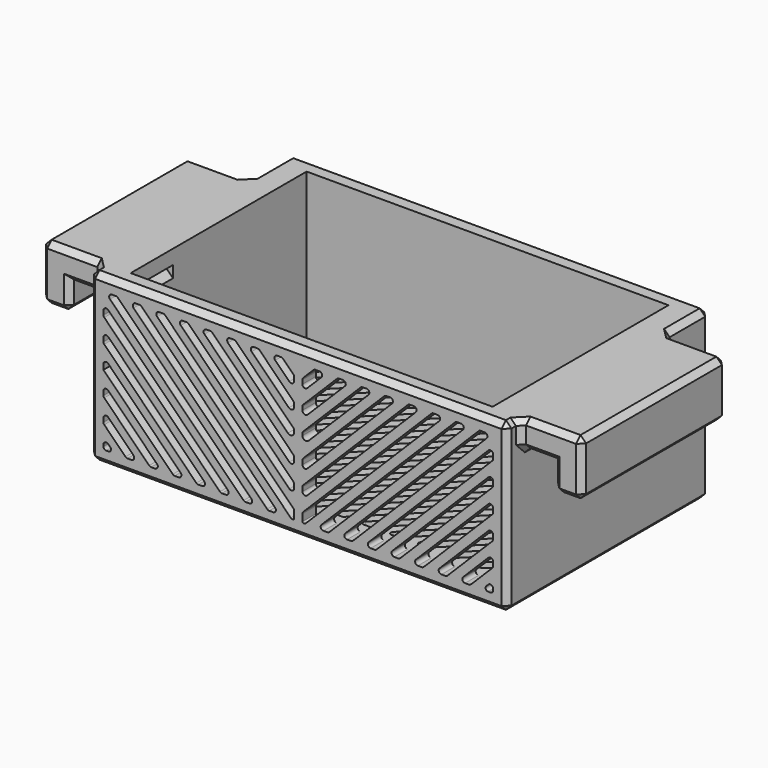
from build123d import *

# Parameters (mm, degrees)
F0_W          = 10
F0_H          = 65
F1_DEPTH      = 10
F1_DEPTH_BACK = 10
F0_W_2        = 12
F2_DEPTH      = 10
F3_DEPTH      = 10
F3_DEPTH_BACK = 50
F4_DEPTH      = 10
F4_DEPTH_BACK = 50
F0_W_3        = 130
F0_H_2        = 6
F5_DEPTH      = 10
F5_DEPTH_BACK = 50
F6_START      = -45
F0_H_3        = 79
F6_DEPTH      = 5
F8_DEPTH      = 58.3
F9_SIZE       = 2
F11_DEPTH     = 25
F12_DEPTH     = 25


with BuildPart() as f1:
    # F0 (on Top) → F1 (new body, two sides)
    with BuildSketch(Plane.XY) as f1_sk:
        with Locations((-167, -32.5)):
            Rectangle(F0_W, F0_H)
    extrude(amount=-F1_DEPTH)
    extrude(f1_sk.sketch, amount=F1_DEPTH_BACK)

    # F0 (on Top) → F2 (join)
    with BuildSketch(Plane.XY):
        with Locations((-156, -32.5)):
            Rectangle(F0_W_2, F0_H)
    extrude(amount=F2_DEPTH)

    # F0 (on Top) → F3 (join, two sides)
    with BuildSketch(Plane.XY) as f3_sk:
        Polygon((-150, -65), (-140, -65), (-140, 14), (-140, 20), (-150, 20), (-150, 0), align=None)
    extrude(amount=F3_DEPTH)
    extrude(f3_sk.sketch, amount=-F3_DEPTH_BACK)



with BuildPart() as f1b:
    # F0 (on Top) → F1, piece 2 (new body, two sides)
    with BuildSketch(Plane.XY) as f1_2_sk:
        with Locations((17, -32.5)):
            Rectangle(F0_W, F0_H)
    extrude(amount=-F1_DEPTH)
    extrude(f1_2_sk.sketch, amount=F1_DEPTH_BACK)

    # F0 (on Top) → F2, piece 2 (join)
    with BuildSketch(Plane.XY):
        with Locations((6, -32.5)):
            Rectangle(F0_W_2, F0_H)
    extrude(amount=F2_DEPTH)

    # F0 (on Top) → F3, piece 2 (join, two sides)
    with BuildSketch(Plane.XY) as f3_2_sk:
        Polygon((0, -65), (0, 0), (0, 20), (-10, 20), (-10, 14), (-10, -65), align=None)
    extrude(amount=F3_DEPTH)
    extrude(f3_2_sk.sketch, amount=-F3_DEPTH_BACK)


with BuildPart() as f1_1:
    add(f1.part)

    add(f1b.part)  # F4 merges F1b
    # F0 (on Top) → F4 (join, two sides)
    with BuildSketch(Plane.XY) as f4_sk:
        Polygon((0, -71), (0, -65), (-10, -65), (-140, -65), (-150, -65), (-150, -71), align=None)
    extrude(amount=F4_DEPTH)
    extrude(f4_sk.sketch, amount=-F4_DEPTH_BACK)

    # F0 (on Top) → F5 (join, two sides)
    with BuildSketch(Plane.XY) as f5_sk:
        with Locations((-75, 17)):
            Rectangle(F0_W_3, F0_H_2)
    extrude(amount=F5_DEPTH)
    extrude(f5_sk.sketch, amount=-F5_DEPTH_BACK)

    # F0 (on Top) → F6 (join)
    with BuildSketch(Plane.XY.offset(F6_START)):
        with Locations((-75, -25.5)):
            Rectangle(F0_W_3, F0_H_3)
    extrude(amount=-F6_DEPTH)

    # F7 (on face) → F8 (cut)
    with BuildSketch(Plane.XY):
        with BuildLine():
            Line((-131, 10), (-136, 5))
            Line((-136, 5), (-136, 2.4142135624))
            ThreePointArc((-136, 2.4142135624), (-135.3826834324, 1.4903340299), (-134.2928932188, 1.7071067812))
            Line((-134.2928932188, 1.7071067812), (-127.7071067812, 8.2928932188))
            ThreePointArc((-127.7071067812, 8.2928932188), (-127.4903340299, 9.3826834324), (-128.4142135624, 10))
            Line((-128.4142135624, 10), (-131, 10))
        make_face()
        with BuildLine():
            Line((-121.2928932188, 9.7071067812), (-135.7071067812, -4.7071067812))
            ThreePointArc((-135.7071067812, -4.7071067812), (-135.9238795325, -5.03153013), (-136, -5.4142135624))
            Line((-136, -5.4142135624), (-136, -7.5857864376))
            ThreePointArc((-136, -7.5857864376), (-135.3826834324, -8.5096659701), (-134.2928932188, -8.2928932188))
            Line((-134.2928932188, -8.2928932188), (-117.7071067812, 8.2928932188))
            ThreePointArc((-117.7071067812, 8.2928932188), (-117.4903340299, 9.3826834324), (-118.4142135624, 10))
            Line((-118.4142135624, 10), (-120.5857864376, 10))
            ThreePointArc((-120.5857864376, 10), (-120.96846987, 9.9238795325), (-121.2928932188, 9.7071067812))
        make_face()
        with BuildLine():
            Line((-111.2928932188, 9.7071067812), (-135.7071067812, -14.7071067812))
            ThreePointArc((-135.7071067812, -14.7071067812), (-135.9238795325, -15.03153013), (-136, -15.4142135624))
            Line((-136, -15.4142135624), (-136, -17.5857864376))
            ThreePointArc((-136, -17.5857864376), (-135.3826834324, -18.5096659701), (-134.2928932188, -18.2928932188))
            Line((-134.2928932188, -18.2928932188), (-107.7071067812, 8.2928932188))
            ThreePointArc((-107.7071067812, 8.2928932188), (-107.4903340299, 9.3826834324), (-108.4142135624, 10))
            Line((-108.4142135624, 10), (-110.5857864376, 10))
            ThreePointArc((-110.5857864376, 10), (-110.96846987, 9.9238795325), (-111.2928932188, 9.7071067812))
        make_face()
        with BuildLine():
            Line((-101.2928932188, 9.7071067812), (-135.7071067812, -24.7071067812))
            ThreePointArc((-135.7071067812, -24.7071067812), (-135.9238795325, -25.03153013), (-136, -25.4142135624))
            Line((-136, -25.4142135624), (-136, -27.5857864376))
            ThreePointArc((-136, -27.5857864376), (-135.3826834324, -28.5096659701), (-134.2928932188, -28.2928932188))
            Line((-134.2928932188, -28.2928932188), (-97.7071067812, 8.2928932188))
            ThreePointArc((-97.7071067812, 8.2928932188), (-97.4903340299, 9.3826834324), (-98.4142135624, 10))
            Line((-98.4142135624, 10), (-100.5857864376, 10))
            ThreePointArc((-100.5857864376, 10), (-100.96846987, 9.9238795325), (-101.2928932188, 9.7071067812))
        make_face()
        with BuildLine():
            Line((-91.2928932188, 9.7071067812), (-135.7071067812, -34.7071067812))
            ThreePointArc((-135.7071067812, -34.7071067812), (-135.9238795325, -35.03153013), (-136, -35.4142135624))
            Line((-136, -35.4142135624), (-136, -37.5857864376))
            ThreePointArc((-136, -37.5857864376), (-135.3826834324, -38.5096659701), (-134.2928932188, -38.2928932188))
            Line((-134.2928932188, -38.2928932188), (-87.7071067812, 8.2928932188))
            ThreePointArc((-87.7071067812, 8.2928932188), (-87.4903340299, 9.3826834324), (-88.4142135624, 10))
            Line((-88.4142135624, 10), (-90.5857864376, 10))
            ThreePointArc((-90.5857864376, 10), (-90.96846987, 9.9238795325), (-91.2928932188, 9.7071067812))
        make_face()
        with BuildLine():
            Line((-81.2928932188, 9.7071067812), (-135.7071067812, -44.7071067812))
            ThreePointArc((-135.7071067812, -44.7071067812), (-135.9238795325, -45.03153013), (-136, -45.4142135624))
            Line((-136, -45.4142135624), (-136, -47.5857864376))
            ThreePointArc((-136, -47.5857864376), (-135.3826834324, -48.5096659701), (-134.2928932188, -48.2928932188))
            Line((-134.2928932188, -48.2928932188), (-77.7071067812, 8.2928932188))
            ThreePointArc((-77.7071067812, 8.2928932188), (-77.4903340299, 9.3826834324), (-78.4142135624, 10))
            Line((-78.4142135624, 10), (-80.5857864376, 10))
            ThreePointArc((-80.5857864376, 10), (-80.96846987, 9.9238795325), (-81.2928932188, 9.7071067812))
        make_face()
        with BuildLine():
            Line((-71.2928932188, 9.7071067812), (-135.7071067812, -54.7071067812))
            ThreePointArc((-135.7071067812, -54.7071067812), (-135.9238795325, -55.03153013), (-136, -55.4142135624))
            Line((-136, -55.4142135624), (-136, -57.5857864376))
            ThreePointArc((-136, -57.5857864376), (-135.3826834324, -58.5096659701), (-134.2928932188, -58.2928932188))
            Line((-134.2928932188, -58.2928932188), (-67.7071067812, 8.2928932188))
            ThreePointArc((-67.7071067812, 8.2928932188), (-67.4903340299, 9.3826834324), (-68.4142135624, 10))
            Line((-68.4142135624, 10), (-70.5857864376, 10))
            ThreePointArc((-70.5857864376, 10), (-70.96846987, 9.9238795325), (-71.2928932188, 9.7071067812))
        make_face()
        with BuildLine():
            ThreePointArc((-130.2928932188, -59.2928932188), (-130.5096659701, -60.3826834324), (-129.5857864376, -61))
            Line((-129.5857864376, -61), (-127.4142135624, -61))
            ThreePointArc((-127.4142135624, -61), (-127.03153013, -60.9238795325), (-126.7071067812, -60.7071067812))
            Line((-126.7071067812, -60.7071067812), (-57.7071067812, 8.2928932188))
            ThreePointArc((-57.7071067812, 8.2928932188), (-57.4903340299, 9.3826834324), (-58.4142135624, 10))
            Line((-58.4142135624, 10), (-60.5857864376, 10))
            ThreePointArc((-60.5857864376, 10), (-60.96846987, 9.9238795325), (-61.2928932188, 9.7071067812))
            Line((-61.2928932188, 9.7071067812), (-130.2928932188, -59.2928932188))
        make_face()
        with BuildLine():
            Line((-51.2928932188, 9.7071067812), (-120.2928932188, -59.2928932188))
            ThreePointArc((-120.2928932188, -59.2928932188), (-120.5096659701, -60.3826834324), (-119.5857864376, -61))
            Line((-119.5857864376, -61), (-117.4142135624, -61))
            ThreePointArc((-117.4142135624, -61), (-117.03153013, -60.9238795325), (-116.7071067812, -60.7071067812))
            Line((-116.7071067812, -60.7071067812), (-47.7071067812, 8.2928932188))
            ThreePointArc((-47.7071067812, 8.2928932188), (-47.4903340299, 9.3826834324), (-48.4142135624, 10))
            Line((-48.4142135624, 10), (-50.5857864376, 10))
            ThreePointArc((-50.5857864376, 10), (-50.96846987, 9.9238795325), (-51.2928932188, 9.7071067812))
        make_face()
        with BuildLine():
            Line((-41.2928932188, 9.7071067812), (-110.2928932188, -59.2928932188))
            ThreePointArc((-110.2928932188, -59.2928932188), (-110.5096659701, -60.3826834324), (-109.5857864376, -61))
            Line((-109.5857864376, -61), (-107.4142135624, -61))
            ThreePointArc((-107.4142135624, -61), (-107.03153013, -60.9238795325), (-106.7071067812, -60.7071067812))
            Line((-106.7071067812, -60.7071067812), (-37.7071067812, 8.2928932188))
            ThreePointArc((-37.7071067812, 8.2928932188), (-37.4903340299, 9.3826834324), (-38.4142135624, 10))
            Line((-38.4142135624, 10), (-40.5857864376, 10))
            ThreePointArc((-40.5857864376, 10), (-40.96846987, 9.9238795325), (-41.2928932188, 9.7071067812))
        make_face()
        with BuildLine():
            Line((-31.2928932188, 9.7071067812), (-100.2928932188, -59.2928932188))
            ThreePointArc((-100.2928932188, -59.2928932188), (-100.5096659701, -60.3826834324), (-99.5857864376, -61))
            Line((-99.5857864376, -61), (-97, -61))
            Line((-97, -61), (-27.7071067812, 8.2928932188))
            ThreePointArc((-27.7071067812, 8.2928932188), (-27.4903340299, 9.3826834324), (-28.4142135624, 10))
            Line((-28.4142135624, 10), (-30.5857864376, 10))
            ThreePointArc((-30.5857864376, 10), (-30.96846987, 9.9238795325), (-31.2928932188, 9.7071067812))
        make_face()
        with BuildLine():
            ThreePointArc((-17.7071067812, 8.2928932188), (-17.4903340299, 9.3826834324), (-18.4142135624, 10))
            Line((-18.4142135624, 10), (-20.5857864376, 10))
            ThreePointArc((-20.5857864376, 10), (-20.96846987, 9.9238795325), (-21.2928932188, 9.7071067812))
            Line((-21.2928932188, 9.7071067812), (-90.2928932188, -59.2928932188))
            ThreePointArc((-90.2928932188, -59.2928932188), (-90.5096659701, -60.3826834324), (-89.5857864376, -61))
            Line((-89.5857864376, -61), (-87.4142135624, -61))
            ThreePointArc((-87.4142135624, -61), (-87.03153013, -60.9238795325), (-86.7071067812, -60.7071067812))
            Line((-86.7071067812, -60.7071067812), (-17.7071067812, 8.2928932188))
        make_face()
        with BuildLine():
            Line((-15.7071067812, 5.2928932188), (-80.2928932188, -59.2928932188))
            ThreePointArc((-80.2928932188, -59.2928932188), (-80.5096659701, -60.3826834324), (-79.5857864376, -61))
            Line((-79.5857864376, -61), (-77.4142135624, -61))
            ThreePointArc((-77.4142135624, -61), (-77.03153013, -60.9238795325), (-76.7071067812, -60.7071067812))
            Line((-76.7071067812, -60.7071067812), (-14.2928932188, 1.7071067812))
            ThreePointArc((-14.2928932188, 1.7071067812), (-14.0761204675, 2.03153013), (-14, 2.4142135624))
            Line((-14, 2.4142135624), (-14, 4.5857864376))
            ThreePointArc((-14, 4.5857864376), (-14.6173165676, 5.5096659701), (-15.7071067812, 5.2928932188))
        make_face()
        with BuildLine():
            Line((-15.7071067812, -4.7071067812), (-70.2928932188, -59.2928932188))
            ThreePointArc((-70.2928932188, -59.2928932188), (-70.5096659701, -60.3826834324), (-69.5857864376, -61))
            Line((-69.5857864376, -61), (-67.4142135624, -61))
            ThreePointArc((-67.4142135624, -61), (-67.03153013, -60.9238795325), (-66.7071067812, -60.7071067812))
            Line((-66.7071067812, -60.7071067812), (-14.2928932188, -8.2928932188))
            ThreePointArc((-14.2928932188, -8.2928932188), (-14.0761204675, -7.96846987), (-14, -7.5857864376))
            Line((-14, -7.5857864376), (-14, -5.4142135624))
            ThreePointArc((-14, -5.4142135624), (-14.6173165676, -4.4903340299), (-15.7071067812, -4.7071067812))
        make_face()
        with BuildLine():
            Line((-15.7071067812, -14.7071067812), (-60.2928932188, -59.2928932188))
            ThreePointArc((-60.2928932188, -59.2928932188), (-60.5096659701, -60.3826834324), (-59.5857864376, -61))
            Line((-59.5857864376, -61), (-57.4142135624, -61))
            ThreePointArc((-57.4142135624, -61), (-57.03153013, -60.9238795325), (-56.7071067812, -60.7071067812))
            Line((-56.7071067812, -60.7071067812), (-14.2928932188, -18.2928932188))
            ThreePointArc((-14.2928932188, -18.2928932188), (-14.0761204675, -17.96846987), (-14, -17.5857864376))
            Line((-14, -17.5857864376), (-14, -15.4142135624))
            ThreePointArc((-14, -15.4142135624), (-14.6173165676, -14.4903340299), (-15.7071067812, -14.7071067812))
        make_face()
        with BuildLine():
            Line((-15.7071067812, -24.7071067812), (-50.2928932188, -59.2928932188))
            ThreePointArc((-50.2928932188, -59.2928932188), (-50.5096659701, -60.3826834324), (-49.5857864376, -61))
            Line((-49.5857864376, -61), (-47.4142135624, -61))
            ThreePointArc((-47.4142135624, -61), (-47.03153013, -60.9238795325), (-46.7071067812, -60.7071067812))
            Line((-46.7071067812, -60.7071067812), (-14.2928932188, -28.2928932188))
            ThreePointArc((-14.2928932188, -28.2928932188), (-14.0761204675, -27.96846987), (-14, -27.5857864376))
            Line((-14, -27.5857864376), (-14, -25.4142135624))
            ThreePointArc((-14, -25.4142135624), (-14.6173165676, -24.4903340299), (-15.7071067812, -24.7071067812))
        make_face()
        with BuildLine():
            Line((-15.7071067812, -34.7071067812), (-40.2928932188, -59.2928932188))
            ThreePointArc((-40.2928932188, -59.2928932188), (-40.5096659701, -60.3826834324), (-39.5857864376, -61))
            Line((-39.5857864376, -61), (-37.4142135624, -61))
            ThreePointArc((-37.4142135624, -61), (-37.03153013, -60.9238795325), (-36.7071067812, -60.7071067812))
            Line((-36.7071067812, -60.7071067812), (-14.2928932188, -38.2928932188))
            ThreePointArc((-14.2928932188, -38.2928932188), (-14.0761204675, -37.96846987), (-14, -37.5857864376))
            Line((-14, -37.5857864376), (-14, -35.4142135624))
            ThreePointArc((-14, -35.4142135624), (-14.6173165676, -34.4903340299), (-15.7071067812, -34.7071067812))
        make_face()
        with BuildLine():
            Line((-15.7071067812, -44.7071067812), (-30.2928932188, -59.2928932188))
            ThreePointArc((-30.2928932188, -59.2928932188), (-30.5096659701, -60.3826834324), (-29.5857864376, -61))
            Line((-29.5857864376, -61), (-27.4142135624, -61))
            ThreePointArc((-27.4142135624, -61), (-27.03153013, -60.9238795325), (-26.7071067812, -60.7071067812))
            Line((-26.7071067812, -60.7071067812), (-14, -48))
            Line((-14, -48), (-14, -45.4142135624))
            ThreePointArc((-14, -45.4142135624), (-14.6173165676, -44.4903340299), (-15.7071067812, -44.7071067812))
        make_face()
        with BuildLine():
            Line((-16.7071067812, -60.7071067812), (-14, -58))
            Line((-14, -58), (-14, -55.4142135624))
            ThreePointArc((-14, -55.4142135624), (-14.6173165676, -54.4903340299), (-15.7071067812, -54.7071067812))
            Line((-15.7071067812, -54.7071067812), (-20.2928932188, -59.2928932188))
            ThreePointArc((-20.2928932188, -59.2928932188), (-20.5096659701, -60.3826834324), (-19.5857864376, -61))
            Line((-19.5857864376, -61), (-17.4142135624, -61))
            ThreePointArc((-17.4142135624, -61), (-17.03153013, -60.9238795325), (-16.7071067812, -60.7071067812))
        make_face()
    extrude(amount=-F8_DEPTH, mode=Mode.SUBTRACT)

    # F9
    f9_edges = [f1_1.edges().sort_by_distance(p)[0] for p in [
        (-156, -65, 0),
        (-156, 0, 0),
        (-172, -65, 0),
        (-161, -65, 10),
        (-150, -65, 5),
        (-162, -65, -5),
        (-167, -65, -10),
        (-162, 0, -5),
        (-167, 0, -10),
        (-172, 0, 0),
        (-161, 0, 10),
        (-150, 0, 5),
        (-162, -32.5, -10),
        (-172, -32.5, -10),
        (12, -65, -5),
        (6, -65, 0),
        (0, -65, 5),
        (11, -65, 10),
        (22, -65, 0),
        (17, -65, -10),
        (17, 0, -10),
        (12, 0, -5),
        (6, 0, 0),
        (0, 0, 5),
        (11, 0, 10),
        (22, 0, 0),
        (12, -32.5, -10),
        (22, -32.5, -10),
        (-150, -71, -20),
        (-75, -71, 10),
        (0, -71, -20),
        (-75, -71, -50),
        (-150, -68, 10),
        (-150, -25.5, -50),
        (-150, 20, -20),
        (-150, 10, 10),
        (-150, -32.5, 0),
        (-75, 20, 10),
        (-75, 20, -50),
        (0, 20, -20),
        (0, -25.5, -50),
        (0, -68, 10),
        (0, -32.5, 0),
        (0, 10, 10),
        (22, -32.5, 10),
        (-172, -32.5, 10),
    ]]
    chamfer(f9_edges, length=F9_SIZE)

    # F10 (on face) → F11 (cut)
    with BuildSketch(Plane.XZ.offset(71)):
        with BuildLine():
            ThreePointArc((-145, -44), (-144.7071067812, -44.7071067812), (-144, -45))
            Line((-144, -45), (-143.1727922061, -45))
            ThreePointArc((-143.1727922061, -45), (-142.3413006269, -44.4444150891), (-142.5363961031, -43.4636038969))
            Line((-142.5363961031, -43.4636038969), (-143.2928932188, -42.7071067812))
            ThreePointArc((-143.2928932188, -42.7071067812), (-144.3826834324, -42.4903340299), (-145, -43.4142135624))
            Line((-145, -43.4142135624), (-145, -44))
        make_face()
        with BuildLine():
            ThreePointArc((-145, -36.3431457505), (-144.9238795325, -36.7258291829), (-144.7071067812, -37.0502525317))
            Line((-144.7071067812, -37.0502525317), (-137.0502525317, -44.7071067812))
            ThreePointArc((-137.0502525317, -44.7071067812), (-136.7258291829, -44.9238795325), (-136.3431457505, -45))
            Line((-136.3431457505, -45), (-134.9342135624, -45))
            ThreePointArc((-134.9342135624, -45), (-134.0103340299, -44.3826834324), (-134.2271067812, -43.2928932188))
            Line((-134.2271067812, -43.2928932188), (-143.2928932188, -34.2271067812))
            ThreePointArc((-143.2928932188, -34.2271067812), (-144.3826834324, -34.0103340299), (-145, -34.9342135624))
            Line((-145, -34.9342135624), (-145, -36.3431457505))
        make_face()
        with BuildLine():
            ThreePointArc((-145, -27.8631457505), (-144.9238795325, -28.2458291829), (-144.7071067812, -28.5702525317))
            Line((-144.7071067812, -28.5702525317), (-128.5702525317, -44.7071067812))
            ThreePointArc((-128.5702525317, -44.7071067812), (-128.2458291829, -44.9238795325), (-127.8631457505, -45))
            Line((-127.8631457505, -45), (-126.4542135624, -45))
            ThreePointArc((-126.4542135624, -45), (-125.5303340299, -44.3826834324), (-125.7471067812, -43.2928932188))
            Line((-125.7471067812, -43.2928932188), (-143.2928932188, -25.7471067812))
            ThreePointArc((-143.2928932188, -25.7471067812), (-144.3826834324, -25.5303340299), (-145, -26.4542135624))
            Line((-145, -26.4542135624), (-145, -27.8631457505))
        make_face()
        with BuildLine():
            Line((-145, -17.9742135624), (-145, -19.7973593129))
            Line((-145, -19.7973593129), (-120.0902525317, -44.7071067812))
            ThreePointArc((-120.0902525317, -44.7071067812), (-119.7658291829, -44.9238795325), (-119.3831457505, -45))
            Line((-119.3831457505, -45), (-117.9742135624, -45))
            ThreePointArc((-117.9742135624, -45), (-117.0503340299, -44.3826834324), (-117.2671067812, -43.2928932188))
            Line((-117.2671067812, -43.2928932188), (-143.2928932188, -17.2671067812))
            ThreePointArc((-143.2928932188, -17.2671067812), (-144.3826834324, -17.0503340299), (-145, -17.9742135624))
        make_face()
        with BuildLine():
            ThreePointArc((-145, -10.9031457505), (-144.9238795325, -11.2858291829), (-144.7071067812, -11.6102525317))
            Line((-144.7071067812, -11.6102525317), (-111.6102525317, -44.7071067812))
            ThreePointArc((-111.6102525317, -44.7071067812), (-111.2858291829, -44.9238795325), (-110.9031457505, -45))
            Line((-110.9031457505, -45), (-109.4942135624, -45))
            ThreePointArc((-109.4942135624, -45), (-108.5703340299, -44.3826834324), (-108.7871067812, -43.2928932188))
            Line((-108.7871067812, -43.2928932188), (-143.2928932188, -8.7871067812))
            ThreePointArc((-143.2928932188, -8.7871067812), (-144.3826834324, -8.5703340299), (-145, -9.4942135624))
            Line((-145, -9.4942135624), (-145, -10.9031457505))
        make_face()
        with BuildLine():
            ThreePointArc((-143.2928932188, -0.3071067812), (-144.3826834324, -0.0903340299), (-145, -1.0142135624))
            Line((-145, -1.0142135624), (-145, -2.4231457505))
            ThreePointArc((-145, -2.4231457505), (-144.9238795325, -2.8058291829), (-144.7071067812, -3.1302525317))
            Line((-144.7071067812, -3.1302525317), (-103.1302525317, -44.7071067812))
            ThreePointArc((-103.1302525317, -44.7071067812), (-102.8058291829, -44.9238795325), (-102.4231457505, -45))
            Line((-102.4231457505, -45), (-101.0142135624, -45))
            ThreePointArc((-101.0142135624, -45), (-100.0903340299, -44.3826834324), (-100.3071067812, -43.2928932188))
            Line((-100.3071067812, -43.2928932188), (-143.2928932188, -0.3071067812))
        make_face()
        with BuildLine():
            ThreePointArc((-141.9431457505, 5), (-142.867025283, 4.3826834324), (-142.6502525317, 3.2928932188))
            Line((-142.6502525317, 3.2928932188), (-94.6502525317, -44.7071067812))
            ThreePointArc((-94.6502525317, -44.7071067812), (-94.3258291829, -44.9238795325), (-93.9431457505, -45))
            Line((-93.9431457505, -45), (-92.5342135624, -45))
            ThreePointArc((-92.5342135624, -45), (-91.6103340299, -44.3826834324), (-91.8271067812, -43.2928932188))
            Line((-91.8271067812, -43.2928932188), (-139.8271067812, 4.7071067812))
            ThreePointArc((-139.8271067812, 4.7071067812), (-140.15153013, 4.9238795325), (-140.5342135624, 5))
            Line((-140.5342135624, 5), (-141.9431457505, 5))
        make_face()
        with BuildLine():
            ThreePointArc((-133.4631457505, 5), (-134.387025283, 4.3826834324), (-134.1702525317, 3.2928932188))
            Line((-134.1702525317, 3.2928932188), (-86.1702525317, -44.7071067812))
            ThreePointArc((-86.1702525317, -44.7071067812), (-85.8458291829, -44.9238795325), (-85.4631457505, -45))
            Line((-85.4631457505, -45), (-84.0542135624, -45))
            ThreePointArc((-84.0542135624, -45), (-83.1303340299, -44.3826834324), (-83.3471067812, -43.2928932188))
            Line((-83.3471067812, -43.2928932188), (-131.3471067812, 4.7071067812))
            ThreePointArc((-131.3471067812, 4.7071067812), (-131.67153013, 4.9238795325), (-132.0542135624, 5))
            Line((-132.0542135624, 5), (-133.4631457505, 5))
        make_face()
        with BuildLine():
            ThreePointArc((-124.9831457505, 5), (-125.907025283, 4.3826834324), (-125.6902525317, 3.2928932188))
            Line((-125.6902525317, 3.2928932188), (-77.6902525317, -44.7071067812))
            ThreePointArc((-77.6902525317, -44.7071067812), (-77.3703853255, -44.9219791275), (-76.9930187911, -44.9999512603))
            ThreePointArc((-76.9930187911, -44.9999512603), (-76.6439869353, -44.8510764842), (-76.5, -44.5))
            Line((-76.5, -44.5), (-76.5, -42.0689321881))
            ThreePointArc((-76.5, -42.0689321881), (-76.5761204675, -41.6862487558), (-76.7928932188, -41.3618254069))
            Line((-76.7928932188, -41.3618254069), (-122.8618254069, 4.7071067812))
            ThreePointArc((-122.8618254069, 4.7071067812), (-123.1862487558, 4.9238795325), (-123.5689321881, 5))
            Line((-123.5689321881, 5), (-124.9831457505, 5))
        make_face()
        with BuildLine():
            ThreePointArc((-116.5031457505, 5), (-117.427025283, 4.3826834324), (-117.2102525317, 3.2928932188))
            Line((-117.2102525317, 3.2928932188), (-78.2071067812, -35.7102525317))
            ThreePointArc((-78.2071067812, -35.7102525317), (-77.1173165676, -35.927025283), (-76.5, -35.0031457505))
            Line((-76.5, -35.0031457505), (-76.5, -33.5889321881))
            ThreePointArc((-76.5, -33.5889321881), (-76.5761204675, -33.2062487558), (-76.7928932188, -32.8818254069))
            Line((-76.7928932188, -32.8818254069), (-114.3818254069, 4.7071067812))
            ThreePointArc((-114.3818254069, 4.7071067812), (-114.7062487558, 4.9238795325), (-115.0889321881, 5))
            Line((-115.0889321881, 5), (-116.5031457505, 5))
        make_face()
        with BuildLine():
            ThreePointArc((-108.0231457505, 5), (-108.947025283, 4.3826834324), (-108.7302525317, 3.2928932188))
            Line((-108.7302525317, 3.2928932188), (-78.2071067812, -27.2302525317))
            ThreePointArc((-78.2071067812, -27.2302525317), (-77.1173165676, -27.447025283), (-76.5, -26.5231457505))
            Line((-76.5, -26.5231457505), (-76.5, -25.1089321881))
            ThreePointArc((-76.5, -25.1089321881), (-76.5761204675, -24.7262487558), (-76.7928932188, -24.4018254069))
            Line((-76.7928932188, -24.4018254069), (-105.9018254069, 4.7071067812))
            ThreePointArc((-105.9018254069, 4.7071067812), (-106.2262487558, 4.9238795325), (-106.6089321881, 5))
            Line((-106.6089321881, 5), (-108.0231457505, 5))
        make_face()
        with BuildLine():
            ThreePointArc((-99.5431457505, 5), (-100.467025283, 4.3826834324), (-100.2502525317, 3.2928932188))
            Line((-100.2502525317, 3.2928932188), (-78.7192388155, -18.2381204973))
            ThreePointArc((-78.7192388155, -18.2381204973), (-77.3025115379, -18.5199250741), (-76.5, -17.3188816818))
            Line((-76.5, -17.3188816818), (-76.5, -16.6289321881))
            ThreePointArc((-76.5, -16.6289321881), (-76.5761204675, -16.2462487558), (-76.7928932188, -15.9218254069))
            Line((-76.7928932188, -15.9218254069), (-97.4218254069, 4.7071067812))
            ThreePointArc((-97.4218254069, 4.7071067812), (-97.7462487558, 4.9238795325), (-98.1289321881, 5))
            Line((-98.1289321881, 5), (-99.5431457505, 5))
        make_face()
        with BuildLine():
            Line((-77.3973593129, -6.8373593129), (-88.9418254069, 4.7071067812))
            ThreePointArc((-88.9418254069, 4.7071067812), (-89.2662487558, 4.9238795325), (-89.6489321881, 5))
            Line((-89.6489321881, 5), (-91.0631457505, 5))
            ThreePointArc((-91.0631457505, 5), (-91.987025283, 4.3826834324), (-91.7702525317, 3.2928932188))
            Line((-91.7702525317, 3.2928932188), (-78.3778174593, -10.0995418536))
            ThreePointArc((-78.3778174593, -10.0995418536), (-77.1790482244, -10.33799188), (-76.5, -9.3217243943))
            Line((-76.5, -9.3217243943), (-76.5, -8.1489321881))
            ThreePointArc((-76.5, -8.1489321881), (-76.5761204675, -7.7662487558), (-76.7928932188, -7.4418254069))
            Line((-76.7928932188, -7.4418254069), (-77.3973593129, -6.8373593129))
        make_face()
        with BuildLine():
            ThreePointArc((-80.4618254069, 4.7071067812), (-80.7862487558, 4.9238795325), (-81.1689321881, 5))
            Line((-81.1689321881, 5), (-82.5831457505, 5))
            ThreePointArc((-82.5831457505, 5), (-83.507025283, 4.3826834324), (-83.2902525317, 3.2928932188))
            Line((-83.2902525317, 3.2928932188), (-78.2071067812, -1.7902525317))
            ThreePointArc((-78.2071067812, -1.7902525317), (-77.1173165676, -2.007025283), (-76.5, -1.0831457505))
            Line((-76.5, -1.0831457505), (-76.5, 0.3310678119))
            ThreePointArc((-76.5, 0.3310678119), (-76.5761204675, 0.7137512442), (-76.7928932188, 1.0381745931))
            Line((-76.7928932188, 1.0381745931), (-80.4618254069, 4.7071067812))
        make_face()
    extrude(amount=-F11_DEPTH, mode=Mode.SUBTRACT)

    # F10 (on face) → F12 (cut)
    with BuildSketch(Plane.XZ.offset(71)):
        with BuildLine():
            ThreePointArc((-7.3497474683, 3.2928932188), (-7.132974717, 4.3826834324), (-8.0568542495, 5))
            Line((-8.0568542495, 5), (-9.4657864376, 5))
            ThreePointArc((-9.4657864376, 5), (-9.84846987, 4.9238795325), (-10.1728932188, 4.7071067812))
            Line((-10.1728932188, 4.7071067812), (-58.1728932188, -43.2928932188))
            ThreePointArc((-58.1728932188, -43.2928932188), (-58.3896659701, -44.3826834324), (-57.4657864376, -45))
            Line((-57.4657864376, -45), (-56.0568542495, -45))
            ThreePointArc((-56.0568542495, -45), (-55.6741708171, -44.9238795325), (-55.3497474683, -44.7071067812))
            Line((-55.3497474683, -44.7071067812), (-7.3497474683, 3.2928932188))
        make_face()
        with BuildLine():
            Line((-5, -2.4231457505), (-5, -1.0142135624))
            ThreePointArc((-5, -1.0142135624), (-5.6173165676, -0.0903340299), (-6.7071067812, -0.3071067812))
            Line((-6.7071067812, -0.3071067812), (-49.6928932188, -43.2928932188))
            ThreePointArc((-49.6928932188, -43.2928932188), (-49.9096659701, -44.3826834324), (-48.9857864376, -45))
            Line((-48.9857864376, -45), (-47.5768542495, -45))
            ThreePointArc((-47.5768542495, -45), (-47.1941708171, -44.9238795325), (-46.8697474683, -44.7071067812))
            Line((-46.8697474683, -44.7071067812), (-5.2928932188, -3.1302525317))
            ThreePointArc((-5.2928932188, -3.1302525317), (-5.0761204675, -2.8058291829), (-5, -2.4231457505))
        make_face()
        with BuildLine():
            ThreePointArc((-15.8297474683, 3.2928932188), (-15.612974717, 4.3826834324), (-16.5368542495, 5))
            Line((-16.5368542495, 5), (-17.9457864376, 5))
            ThreePointArc((-17.9457864376, 5), (-18.32846987, 4.9238795325), (-18.6528932188, 4.7071067812))
            Line((-18.6528932188, 4.7071067812), (-66.6528932188, -43.2928932188))
            ThreePointArc((-66.6528932188, -43.2928932188), (-66.8696659701, -44.3826834324), (-65.9457864376, -45))
            Line((-65.9457864376, -45), (-64.5368542495, -45))
            ThreePointArc((-64.5368542495, -45), (-64.1541708171, -44.9238795325), (-63.8297474683, -44.7071067812))
            Line((-63.8297474683, -44.7071067812), (-15.8297474683, 3.2928932188))
        make_face()
        with BuildLine():
            Line((-5, -10.9031457505), (-5, -9.4942135624))
            ThreePointArc((-5, -9.4942135624), (-5.6173165676, -8.5703340299), (-6.7071067812, -8.7871067812))
            Line((-6.7071067812, -8.7871067812), (-41.2128932188, -43.2928932188))
            ThreePointArc((-41.2128932188, -43.2928932188), (-41.4296659701, -44.3826834324), (-40.5057864376, -45))
            Line((-40.5057864376, -45), (-39.0968542495, -45))
            ThreePointArc((-39.0968542495, -45), (-38.7141708171, -44.9238795325), (-38.3897474683, -44.7071067812))
            Line((-38.3897474683, -44.7071067812), (-5.2928932188, -11.6102525317))
            ThreePointArc((-5.2928932188, -11.6102525317), (-5.0761204675, -11.2858291829), (-5, -10.9031457505))
        make_face()
        with BuildLine():
            ThreePointArc((-24.3097474683, 3.2928932188), (-24.092974717, 4.3826834324), (-25.0168542495, 5))
            Line((-25.0168542495, 5), (-26.4310678119, 5))
            ThreePointArc((-26.4310678119, 5), (-26.8137512442, 4.9238795325), (-27.1381745931, 4.7071067812))
            Line((-27.1381745931, 4.7071067812), (-73.2071067812, -41.3618254069))
            ThreePointArc((-73.2071067812, -41.3618254069), (-73.4238795325, -41.6862487558), (-73.5, -42.0689321881))
            Line((-73.5, -42.0689321881), (-73.5, -44.5))
            ThreePointArc((-73.5, -44.5), (-73.3560130647, -44.8510764842), (-73.0069812089, -44.9999512603))
            ThreePointArc((-73.0069812089, -44.9999512603), (-72.6296146745, -44.9219791275), (-72.3097474683, -44.7071067812))
            Line((-72.3097474683, -44.7071067812), (-24.3097474683, 3.2928932188))
        make_face()
        with BuildLine():
            Line((-5, -19.7973593129), (-5, -17.9742135624))
            ThreePointArc((-5, -17.9742135624), (-5.6173165676, -17.0503340299), (-6.7071067812, -17.2671067812))
            Line((-6.7071067812, -17.2671067812), (-32.7328932188, -43.2928932188))
            ThreePointArc((-32.7328932188, -43.2928932188), (-32.9496659701, -44.3826834324), (-32.0257864376, -45))
            Line((-32.0257864376, -45), (-30.6168542495, -45))
            ThreePointArc((-30.6168542495, -45), (-30.2341708171, -44.9238795325), (-29.9097474683, -44.7071067812))
            Line((-29.9097474683, -44.7071067812), (-5, -19.7973593129))
        make_face()
        with BuildLine():
            ThreePointArc((-32.7897474683, 3.2928932188), (-32.572974717, 4.3826834324), (-33.4968542495, 5))
            Line((-33.4968542495, 5), (-34.9110678119, 5))
            ThreePointArc((-34.9110678119, 5), (-35.2937512442, 4.9238795325), (-35.6181745931, 4.7071067812))
            Line((-35.6181745931, 4.7071067812), (-73.2071067812, -32.8818254069))
            ThreePointArc((-73.2071067812, -32.8818254069), (-73.4238795325, -33.2062487558), (-73.5, -33.5889321881))
            Line((-73.5, -33.5889321881), (-73.5, -35.0031457505))
            ThreePointArc((-73.5, -35.0031457505), (-72.8826834324, -35.927025283), (-71.7928932188, -35.7102525317))
            Line((-71.7928932188, -35.7102525317), (-32.7897474683, 3.2928932188))
        make_face()
        with BuildLine():
            Line((-5, -27.8631457505), (-5, -26.4542135624))
            ThreePointArc((-5, -26.4542135624), (-5.6173165676, -25.5303340299), (-6.7071067812, -25.7471067812))
            Line((-6.7071067812, -25.7471067812), (-24.2528932188, -43.2928932188))
            ThreePointArc((-24.2528932188, -43.2928932188), (-24.4696659701, -44.3826834324), (-23.5457864376, -45))
            Line((-23.5457864376, -45), (-22.1368542495, -45))
            ThreePointArc((-22.1368542495, -45), (-21.7541708171, -44.9238795325), (-21.4297474683, -44.7071067812))
            Line((-21.4297474683, -44.7071067812), (-5.2928932188, -28.5702525317))
            ThreePointArc((-5.2928932188, -28.5702525317), (-5.0761204675, -28.2458291829), (-5, -27.8631457505))
        make_face()
        with BuildLine():
            ThreePointArc((-41.2697474683, 3.2928932188), (-41.052974717, 4.3826834324), (-41.9768542495, 5))
            Line((-41.9768542495, 5), (-43.3910678119, 5))
            ThreePointArc((-43.3910678119, 5), (-43.7737512442, 4.9238795325), (-44.0981745931, 4.7071067812))
            Line((-44.0981745931, 4.7071067812), (-73.2071067812, -24.4018254069))
            ThreePointArc((-73.2071067812, -24.4018254069), (-73.4238795325, -24.7262487558), (-73.5, -25.1089321881))
            Line((-73.5, -25.1089321881), (-73.5, -26.5231457505))
            ThreePointArc((-73.5, -26.5231457505), (-72.8826834324, -27.447025283), (-71.7928932188, -27.2302525317))
            Line((-71.7928932188, -27.2302525317), (-41.2697474683, 3.2928932188))
        make_face()
        with BuildLine():
            Line((-5, -36.3431457505), (-5, -34.9342135624))
            ThreePointArc((-5, -34.9342135624), (-5.6173165676, -34.0103340299), (-6.7071067812, -34.2271067812))
            Line((-6.7071067812, -34.2271067812), (-15.7728932188, -43.2928932188))
            ThreePointArc((-15.7728932188, -43.2928932188), (-15.9896659701, -44.3826834324), (-15.0657864376, -45))
            Line((-15.0657864376, -45), (-13.6568542495, -45))
            ThreePointArc((-13.6568542495, -45), (-13.2741708171, -44.9238795325), (-12.9497474683, -44.7071067812))
            Line((-12.9497474683, -44.7071067812), (-5.2928932188, -37.0502525317))
            ThreePointArc((-5.2928932188, -37.0502525317), (-5.0761204675, -36.7258291829), (-5, -36.3431457505))
        make_face()
        with BuildLine():
            ThreePointArc((-49.7497474683, 3.2928932188), (-49.532974717, 4.3826834324), (-50.4568542495, 5))
            Line((-50.4568542495, 5), (-51.8710678119, 5))
            ThreePointArc((-51.8710678119, 5), (-52.2537512442, 4.9238795325), (-52.5781745931, 4.7071067812))
            Line((-52.5781745931, 4.7071067812), (-73.2071067812, -15.9218254069))
            ThreePointArc((-73.2071067812, -15.9218254069), (-73.4238795325, -16.2462487558), (-73.5, -16.6289321881))
            Line((-73.5, -16.6289321881), (-73.5, -17.3188816818))
            ThreePointArc((-73.5, -17.3188816818), (-72.6974884621, -18.5199250741), (-71.2807611845, -18.2381204973))
            Line((-71.2807611845, -18.2381204973), (-49.7497474683, 3.2928932188))
        make_face()
        with BuildLine():
            Line((-5, -44), (-5, -43.4142135624))
            ThreePointArc((-5, -43.4142135624), (-5.6173165676, -42.4903340299), (-6.7071067812, -42.7071067812))
            Line((-6.7071067812, -42.7071067812), (-7.4636038969, -43.4636038969))
            ThreePointArc((-7.4636038969, -43.4636038969), (-7.6586993731, -44.4444150891), (-6.8272077939, -45))
            Line((-6.8272077939, -45), (-6, -45))
            ThreePointArc((-6, -45), (-5.2928932188, -44.7071067812), (-5, -44))
        make_face()
        with BuildLine():
            ThreePointArc((-58.2297474683, 3.2928932188), (-58.012974717, 4.3826834324), (-58.9368542495, 5))
            Line((-58.9368542495, 5), (-60.3510678119, 5))
            ThreePointArc((-60.3510678119, 5), (-60.7337512442, 4.9238795325), (-61.0581745931, 4.7071067812))
            Line((-61.0581745931, 4.7071067812), (-72.6026406871, -6.8373593129))
            Line((-72.6026406871, -6.8373593129), (-73.2071067812, -7.4418254069))
            ThreePointArc((-73.2071067812, -7.4418254069), (-73.4238795325, -7.7662487558), (-73.5, -8.1489321881))
            Line((-73.5, -8.1489321881), (-73.5, -9.3217243943))
            ThreePointArc((-73.5, -9.3217243943), (-72.8209517756, -10.33799188), (-71.6221825407, -10.0995418536))
            Line((-71.6221825407, -10.0995418536), (-58.2297474683, 3.2928932188))
        make_face()
        with BuildLine():
            ThreePointArc((-66.7097474683, 3.2928932188), (-66.492974717, 4.3826834324), (-67.4168542495, 5))
            Line((-67.4168542495, 5), (-68.8310678119, 5))
            ThreePointArc((-68.8310678119, 5), (-69.2137512442, 4.9238795325), (-69.5381745931, 4.7071067812))
            Line((-69.5381745931, 4.7071067812), (-73.2071067812, 1.0381745931))
            ThreePointArc((-73.2071067812, 1.0381745931), (-73.4238795325, 0.7137512442), (-73.5, 0.3310678119))
            Line((-73.5, 0.3310678119), (-73.5, -1.0831457505))
            ThreePointArc((-73.5, -1.0831457505), (-72.8826834324, -2.007025283), (-71.7928932188, -1.7902525317))
            Line((-71.7928932188, -1.7902525317), (-66.7097474683, 3.2928932188))
        make_face()
    extrude(amount=-F12_DEPTH, mode=Mode.SUBTRACT)


solid = f1_1.part
